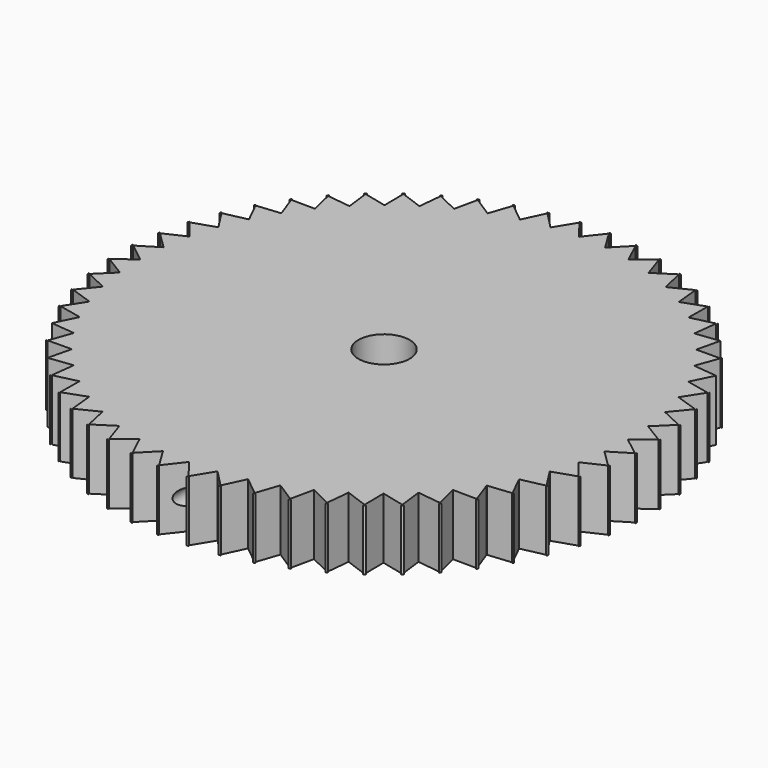
from build123d import *

# Parameters (mm, degrees)
F0_R             = 41.275
F1_DEPTH         = 9.525
F3_DEPTH         = 25.4
F3_COPIES_COUNT  = 14
F3_COPIES_ANGLE  = 83.5714285714
F3_COPIES1_COUNT = 43
F3_COPIES1_ANGLE = 270
F4_R             = 4.0005
F5_DEPTH         = 25.4
F7_DEPTH         = 40.1828


# Not quite as in the source:
# - a pattern or mirror of a feature is missing from the dataset's text; its kind, count and spacing are read off the source's solid


with BuildPart() as f1:
    # F0 (on Top) → F1 (new body)
    with BuildSketch(Plane.XY):
        Circle(F0_R)
    extrude(amount=F1_DEPTH)

    # F2 (on face) → F3 (cut)
    with BuildSketch(Plane.XY.offset(9.525)):
        with BuildLine():
            Line((-41.1851832389, -2.4219615904), (-38.0999972076, -0.0145869281))
            ThreePointArc((-38.0999972076, -0.0145869281), (-38.1, 0), (-38.0999972076, 0.0145869281))
            Line((-38.0999972076, 0.0145869281), (-41.1851832389, 2.4219615904))
            ThreePointArc((-41.1851832389, 2.4219615904), (-41.2025221392, 2.2869910877), (-41.2188666292, 2.151896559))
            ThreePointArc((-41.2188666292, 2.151896559), (-41.275, 0), (-41.2188666292, -2.151896559))
            ThreePointArc((-41.2188666292, -2.151896559), (-41.2025221392, -2.2869910877), (-41.1851832389, -2.4219615904))
        make_face()
    f3 = extrude(amount=-F3_DEPTH, mode=Mode.SUBTRACT)

    # F3_copies: F3 ×14 about axis
    f3_copies_axis = Axis((0, 0, 0), (0, 0, 1))
    for i in range(1, F3_COPIES_COUNT):
        add(f3.rotate(f3_copies_axis, i * F3_COPIES_ANGLE / (F3_COPIES_COUNT - 1)), mode=Mode.SUBTRACT)

    # F3_copies1: F3 ×43 about axis
    f3_copies1_axis = Axis((0, 0, 0), (0, 0, -1))
    for i in range(1, F3_COPIES1_COUNT):
        add(f3.rotate(f3_copies1_axis, i * F3_COPIES1_ANGLE / (F3_COPIES1_COUNT - 1)), mode=Mode.SUBTRACT)

    # F4 (on face) → F5 (cut)
    with BuildSketch(Plane.XY.offset(9.525)):
        Circle(F4_R)
    extrude(amount=-F5_DEPTH, mode=Mode.SUBTRACT)

    # F6 (on Front) → F7 (cut, symmetric)
    with BuildSketch(Plane.XZ):
        with BuildLine():
            ThreePointArc((0, 3.4925), (0.8980256121, 3.8644743879), (1.27, 4.7625))
            ThreePointArc((1.27, 4.7625), (-0.8980256121, 5.6605256121), (0, 3.4925))
        make_face()
    extrude(amount=F7_DEPTH, both=True, mode=Mode.SUBTRACT)


solid = f1.part
